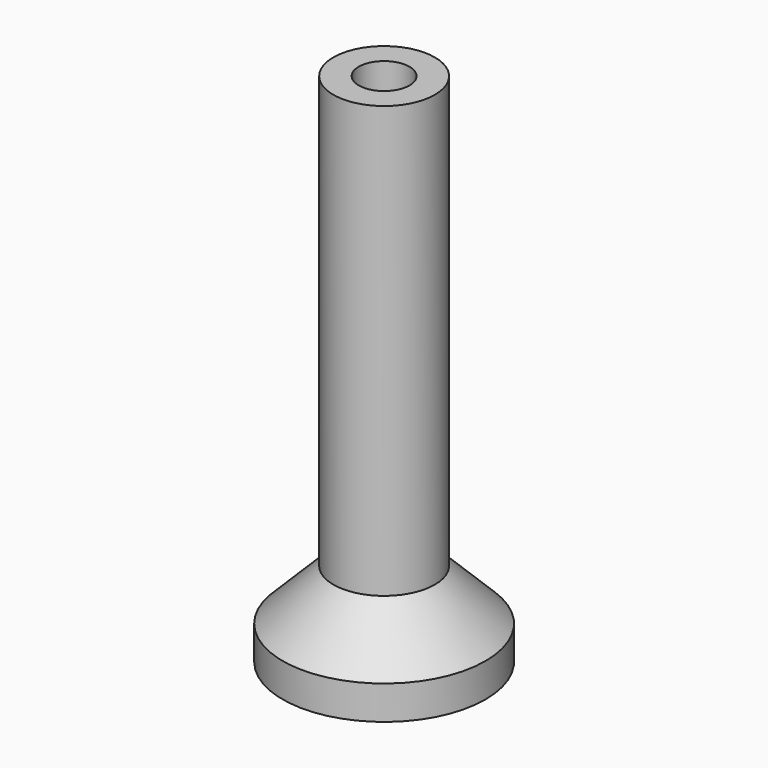
from build123d import *

# Parameters (mm, degrees)
F0_R     = 6
F0_R_2   = 3
F1_DEPTH = 2
F0_R_3   = 1.5
F2_DEPTH = 4
F4_DEPTH = 30.5
F5_SIZE  = 2.99999


# Not quite as in the source:
# - a fillet or chamfer is up to 0.001 mm smaller than in the source, because OpenCascade refuses the exact size


with BuildPart() as f1:
    # F0 (on Top) → F1 (new body)
    with BuildSketch(Plane.XY):
        Circle(F0_R)
        Circle(F0_R_2, mode=Mode.SUBTRACT)
    extrude(amount=F1_DEPTH)



with BuildPart() as f2:
    # F0 (on Top) → F2 (new body)
    with BuildSketch(Plane.XY):
        Circle(F0_R_3)
    extrude(amount=F2_DEPTH)


with BuildPart() as f1_1:
    add(f1.part)

    add(f2.part)  # F4 merges F2
    # F0 (on Top) → F4 (join)
    with BuildSketch(Plane.XY):
        Circle(F0_R_2)
        Circle(F0_R_3, mode=Mode.SUBTRACT)
    extrude(amount=F4_DEPTH)

    # F5 (size 3 in the source; OpenCascade refuses exactly that, so slightly less here)
    f5_edges = [f1_1.edges().sort_by_distance(p)[0] for p in [
        (-3, 0, 2),
    ]]
    chamfer(f5_edges, length=F5_SIZE)


solid = f1_1.part
